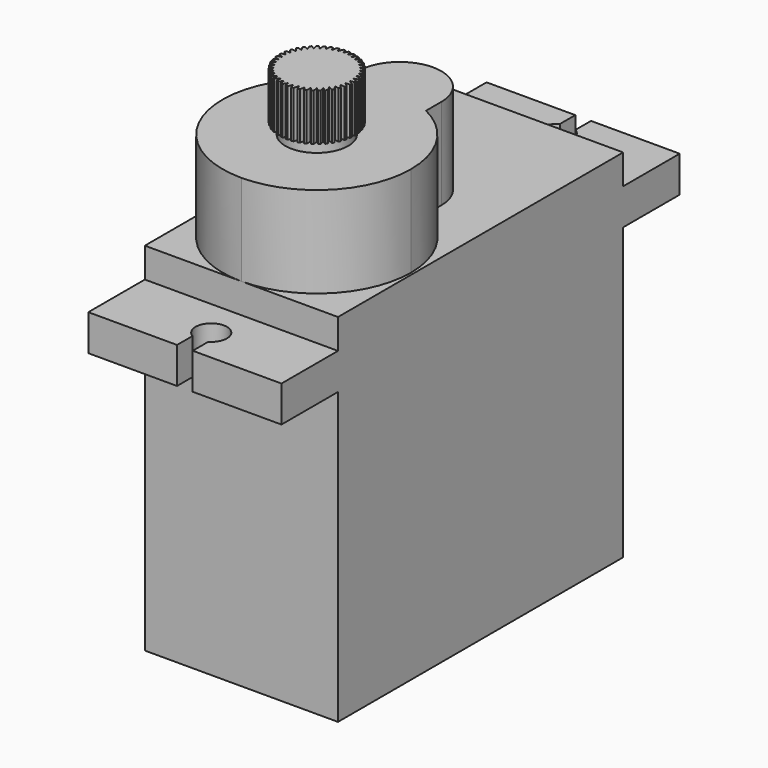
from build123d import *

# Parameters (mm, degrees)
F1_W      = 12.3
F1_H      = 18.5
F2_DEPTH  = 22.7
F3_W      = 12.3
F3_H      = 22.7
F3_H_2    = 4.5
F3_R      = 1
F4_DEPTH  = 2.3
F5_W      = 1
F5_H      = 3.3
F6_DEPTH  = 20.801
F7_W      = 12.3
F7_H      = 22.7
F8_DEPTH  = 1.9
F10_DEPTH = 5.8
F11_R     = 2
F12_DEPTH = 0.7
F13_R     = 2.4
F13_R_2   = 2
F14_DEPTH = 3
F16_DEPTH = 3.7
F17_COUNT = 43


# Not quite as in the source:
# - a feature names something its author has since deleted; it is built from what else it names


with BuildPart() as f2:
    # F1 (on offset) → F2 (new body)
    with BuildSketch(Plane.XZ.offset(70)):
        Rectangle(F1_W, F1_H)
    extrude(amount=F2_DEPTH)

    # F3 (on face) → F4 (join)
    with BuildSketch(Plane.XY.offset(9.25)):
        with Locations((0, -81.35)):
            Rectangle(F3_W, F3_H)
        with Locations((0, -67.75)):
            Rectangle(F3_W, F3_H_2)
        with Locations((0, -67.6)):
            Circle(F3_R, mode=Mode.SUBTRACT)
        with Locations((0, -94.95)):
            Rectangle(F3_W, F3_H_2)
        with Locations((0, -95.1)):
            Circle(F3_R, mode=Mode.SUBTRACT)
    extrude(amount=F4_DEPTH)

    # F5 (on face) → F6 (cut, through all)
    with BuildSketch(Plane.XY.offset(11.55)):
        with Locations((0, -65.5)):
            Rectangle(F5_W, F5_H)
        with Locations((0, -97.2)):
            Rectangle(F5_W, F5_H)
    extrude(amount=-F6_DEPTH, mode=Mode.SUBTRACT)

    # F7 (on face) → F8 (join)
    with BuildSketch(Plane.XY.offset(11.55)):
        with Locations((0, -81.35)):
            Rectangle(F7_W, F7_H)
    extrude(amount=F8_DEPTH)

    # F9 (on face) → F10 (join)
    with BuildSketch(Plane.XY.offset(13.45)):
        with BuildLine():
            ThreePointArc((0, -92.7), (4.2426406871, -90.9426406871), (6, -86.7))
            ThreePointArc((6, -86.7), (5.0941142508, -83.5298265032), (2.65, -81.3169246708))
            ThreePointArc((2.65, -81.3169246708), (0, -80.7), (-2.65, -81.3169246708))
            ThreePointArc((-2.65, -81.3169246708), (-5.843733908, -88.0604315537), (0, -92.7))
        make_face()
        with BuildLine():
            ThreePointArc((-2.65, -81.3169246708), (0, -80.7), (2.65, -81.3169246708))
            Line((2.65, -81.3169246708), (2.65, -80.1))
            ThreePointArc((2.65, -80.1), (0, -77.45), (-2.65, -80.1))
            Line((-2.65, -80.1), (-2.65, -81.3169246708))
        make_face()
    extrude(amount=F10_DEPTH)



with BuildPart() as f12:
    # F11 (on face) → F12 (new body)
    with BuildSketch(Plane.XY.offset(19.25)):
        with Locations((0, -86.7)):
            Circle(F11_R)
    extrude(amount=F12_DEPTH)


with BuildPart() as f2_1:
    add(f2.part)

    add(f12.part)  # F14 merges F12
    # F13 (on face) → F14 (join)
    with BuildSketch(Plane.XY.offset(19.95)):
        with Locations((0, -86.7)):
            Circle(F13_R)
        with Locations((0, -86.7)):
            Circle(F13_R_2, mode=Mode.SUBTRACT)
        with Locations((0, -86.7)):
            Circle(F13_R_2)
    extrude(amount=F14_DEPTH)

    # F17: F16 ×43 about axis
    f17_axis = Axis((0, -86.7, 22.95), (0, 0, 1))


with BuildPart() as f16:
    # F15 (on face) → F16 (new body, through all)
    with BuildSketch(Plane.XY.offset(22.95)):
        with BuildLine():
            ThreePointArc((1.4170132697, -84.7629730529), (1.3273305991, -84.7004516808), (1.2348937398, -84.6420793379))
            Line((1.2348937398, -84.6420793379), (1.1339585762, -84.9085450172))
            Line((1.1339585762, -84.9085450172), (1.4170132697, -84.7629730529))
        make_face()
    extrude(amount=-F16_DEPTH)


with BuildPart() as f2_2:
    add(f2_1.part)
    for i in range(1, F17_COUNT):
        add(f16.part.rotate(f17_axis, i * 360 / F17_COUNT), mode=Mode.SUBTRACT)

    # F17#seed: cut F16
    add(f16.part, mode=Mode.SUBTRACT)


solid = f2_2.part
